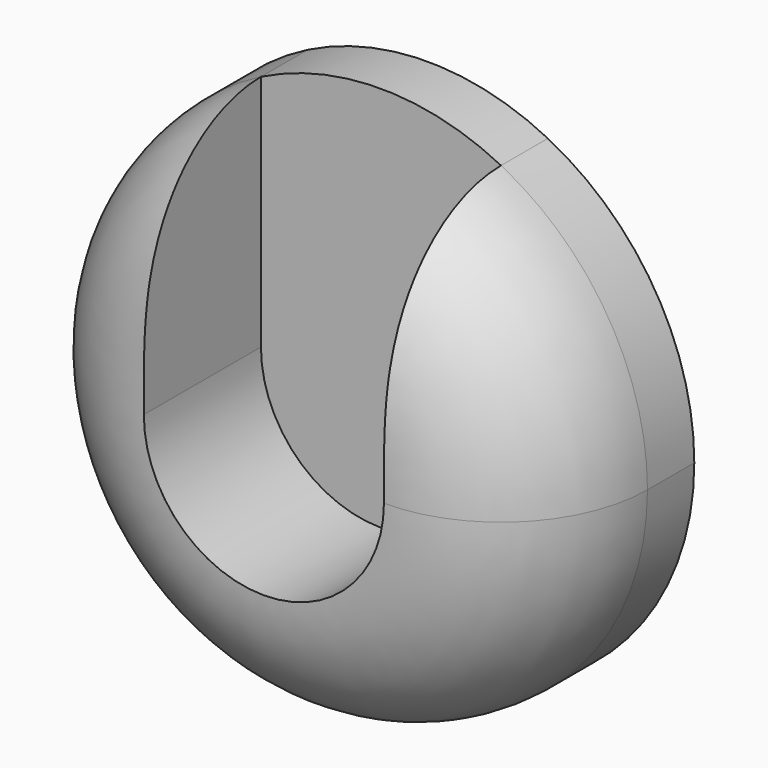
from build123d import *

# Parameters (mm, degrees)
F1_DEPTH = 2
F2_DEPTH = 5
F3_R     = 4.99999


# Not quite as in the source:
# - a fillet or chamfer is up to 0.001 mm smaller than in the source, because OpenCascade refuses the exact size


with BuildPart() as f1:
    # F0 (on Front) → F1 (new body)
    with BuildSketch(Plane.XZ):
        with BuildLine():
            ThreePointArc((-4.1, 8.1240384046), (-4.7696960071, -7.749838708), (9.1, 0))
            ThreePointArc((9.1, 0), (7.749838708, 4.7696960071), (4.1, 8.1240384046))
            Line((4.1, 8.1240384046), (4.1, 0))
            ThreePointArc((4.1, 0), (0, -4.1), (-4.1, 0))
            Line((-4.1, 0), (-4.1, 8.1240384046))
        make_face()
        with BuildLine():
            Line((4.1, 0), (4.1, 8.1240384046))
            ThreePointArc((4.1, 8.1240384046), (0, 9.1), (-4.1, 8.1240384046))
            Line((-4.1, 8.1240384046), (-4.1, 0))
            ThreePointArc((-4.1, 0), (0, -4.1), (4.1, 0))
        make_face()
    extrude(amount=-F1_DEPTH)

    # F0 (on Front) → F2 (join)
    with BuildSketch(Plane.XZ):
        with BuildLine():
            ThreePointArc((-4.1, 8.1240384046), (-4.7696960071, -7.749838708), (9.1, 0))
            ThreePointArc((9.1, 0), (7.749838708, 4.7696960071), (4.1, 8.1240384046))
            Line((4.1, 8.1240384046), (4.1, 0))
            ThreePointArc((4.1, 0), (0, -4.1), (-4.1, 0))
            Line((-4.1, 0), (-4.1, 8.1240384046))
        make_face()
    extrude(amount=F2_DEPTH)

    # F3 (radius 5 in the source; OpenCascade refuses exactly that, so slightly less here)
    f3_edges = [f1.edges().sort_by_distance(p)[0] for p in [
        (-4.769696, -5, -7.749839),
    ]]
    fillet(f3_edges, radius=F3_R)


solid = f1.part
